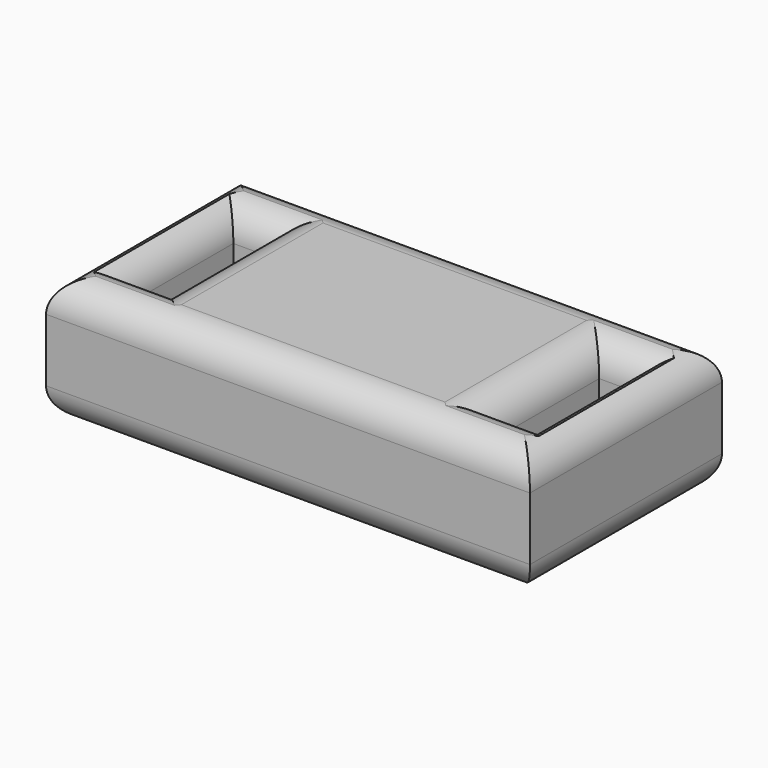
from build123d import *

# Parameters (mm, degrees)
F0_W          = 30.75
F0_H          = 15.25
F0_W_2        = 2.5
F0_H_2        = 8.25
F1_DEPTH      = 8
F2_T1_DEPTH   = 40.75
F2_T3_DEPTH   = 25.25
F2_T5_DEPTH   = 2.5
F2_T7_DEPTH   = 8.25
F2_T9_DEPTH   = 2.5
F2_T15_DEPTH  = 7.5
F2_T20_DEPTH  = 13.25
F2_T28_DEPTH  = 7.5
F2_T32_DEPTH  = 13.25
F2_T40_DEPTH  = 13.25
F2_T45_DEPTH  = 7.5
F2_T52_DEPTH  = 7.5
F2_T57_DEPTH  = 13.25
F2_T65_DEPTH  = 13.25
F2_T70_DEPTH  = 7.5
F2_T77_DEPTH  = 13.25
F2_T82_DEPTH  = 7.5
F2_T89_DEPTH  = 7.5
F2_T94_DEPTH  = 13.25
F2_T102_DEPTH = 13.25
F2_T107_DEPTH = 7.5
F2_T115_DEPTH = 7.5
F2_T120_DEPTH = 13.25
F2_T128_DEPTH = 7.5
F2_T132_DEPTH = 13.25
F2_T140_DEPTH = 13.25
F2_T145_DEPTH = 7.5
F2_T152_DEPTH = 7.5
F2_T157_DEPTH = 13.25
F2_T165_DEPTH = 13.25
F2_T170_DEPTH = 7.5
F2_T177_DEPTH = 13.25
F2_T182_DEPTH = 7.5
F2_T189_DEPTH = 7.5
F2_T194_DEPTH = 13.25
F2_T202_DEPTH = 13.25
F2_T207_DEPTH = 7.5


# Not quite as in the source:
# - a fillet or chamfer that OpenCascade refuses, or shapes differently, is made with other operations: its cross-section is extruded or revolved along the edge and cut away or added


with BuildPart() as f1:
    # F0 (on Top) → F1 (new body)
    with BuildSketch(Plane.XY):
        Rectangle(F0_W, F0_H)
        with Locations((-11.625, 0)):
            Rectangle(F0_W_2, F0_H_2, mode=Mode.SUBTRACT)
        with Locations((11.625, 0)):
            Rectangle(F0_W_2, F0_H_2, mode=Mode.SUBTRACT)
    extrude(amount=F1_DEPTH)

    # F2: fillet of radius 2 on 24 edges, made by hand

    # F2_s2 → F2_t1 (cut)
    with BuildSketch(Plane.YZ.offset(-20.375)):
        with BuildLine():
            ThreePointArc((7.625, 6), (7.0392135624, 7.4142135624), (5.625, 8))
            Line((5.625, 8), (7.625, 8))
            Line((7.625, 8), (7.625, 6))
        make_face()
        with BuildLine():
            ThreePointArc((-7.625, 6), (-7.0392135624, 7.4142135624), (-5.625, 8))
            Line((-5.625, 8), (-7.625, 8))
            Line((-7.625, 8), (-7.625, 6))
        make_face()
        with BuildLine():
            ThreePointArc((7.625, 2), (7.0392135624, 0.5857864376), (5.625, 0))
            Line((5.625, 0), (7.625, 0))
            Line((7.625, 0), (7.625, 2))
        make_face()
        with BuildLine():
            ThreePointArc((-7.625, 2), (-7.0392135624, 0.5857864376), (-5.625, 0))
            Line((-5.625, 0), (-7.625, 0))
            Line((-7.625, 0), (-7.625, 2))
        make_face()
    extrude(amount=F2_T1_DEPTH, mode=Mode.SUBTRACT)

    # F2_s4 → F2_t3 (cut)
    with BuildSketch(Plane.XZ.offset(-12.625)):
        with BuildLine():
            ThreePointArc((-15.375, 6), (-14.7892135624, 7.4142135624), (-13.375, 8))
            Line((-13.375, 8), (-15.375, 8))
            Line((-15.375, 8), (-15.375, 6))
        make_face()
        with BuildLine():
            ThreePointArc((15.375, 6), (14.7892135624, 7.4142135624), (13.375, 8))
            Line((13.375, 8), (15.375, 8))
            Line((15.375, 8), (15.375, 6))
        make_face()
        with BuildLine():
            ThreePointArc((-15.375, 2), (-14.7892135624, 0.5857864376), (-13.375, 0))
            Line((-13.375, 0), (-15.375, 0))
            Line((-15.375, 0), (-15.375, 2))
        make_face()
        with BuildLine():
            ThreePointArc((15.375, 2), (14.7892135624, 0.5857864376), (13.375, 0))
            Line((13.375, 0), (15.375, 0))
            Line((15.375, 0), (15.375, 2))
        make_face()
    extrude(amount=F2_T3_DEPTH, mode=Mode.SUBTRACT)

    # F2_s6 → F2_t5 (cut)
    with BuildSketch(Plane.YZ.offset(-12.875)):
        with BuildLine():
            ThreePointArc((4.125, 6), (4.7107864376, 7.4142135624), (6.125, 8))
            Line((6.125, 8), (4.125, 8))
            Line((4.125, 8), (4.125, 6))
        make_face()
        with BuildLine():
            ThreePointArc((-4.125, 6), (-4.7107864376, 7.4142135624), (-6.125, 8))
            Line((-6.125, 8), (-4.125, 8))
            Line((-4.125, 8), (-4.125, 6))
        make_face()
        with BuildLine():
            ThreePointArc((4.125, 2), (4.7107864376, 0.5857864376), (6.125, 0))
            Line((6.125, 0), (4.125, 0))
            Line((4.125, 0), (4.125, 2))
        make_face()
        with BuildLine():
            ThreePointArc((-4.125, 2), (-4.7107864376, 0.5857864376), (-6.125, 0))
            Line((-6.125, 0), (-4.125, 0))
            Line((-4.125, 0), (-4.125, 2))
        make_face()
    extrude(amount=F2_T5_DEPTH, mode=Mode.SUBTRACT)

    # F2_s8 → F2_t7 (cut)
    with BuildSketch(Plane.XZ.offset(-4.125)):
        with BuildLine():
            ThreePointArc((-10.375, 6), (-9.7892135624, 7.4142135624), (-8.375, 8))
            Line((-8.375, 8), (-10.375, 8))
            Line((-10.375, 8), (-10.375, 6))
        make_face()
        with BuildLine():
            ThreePointArc((-12.875, 6), (-13.4607864376, 7.4142135624), (-14.875, 8))
            Line((-14.875, 8), (-12.875, 8))
            Line((-12.875, 8), (-12.875, 6))
        make_face()
        with BuildLine():
            ThreePointArc((10.375, 6), (9.7892135624, 7.4142135624), (8.375, 8))
            Line((8.375, 8), (10.375, 8))
            Line((10.375, 8), (10.375, 6))
        make_face()
        with BuildLine():
            ThreePointArc((12.875, 6), (13.4607864376, 7.4142135624), (14.875, 8))
            Line((14.875, 8), (12.875, 8))
            Line((12.875, 8), (12.875, 6))
        make_face()
        with BuildLine():
            ThreePointArc((-10.375, 2), (-9.7892135624, 0.5857864376), (-8.375, 0))
            Line((-8.375, 0), (-10.375, 0))
            Line((-10.375, 0), (-10.375, 2))
        make_face()
        with BuildLine():
            ThreePointArc((-12.875, 2), (-13.4607864376, 0.5857864376), (-14.875, 0))
            Line((-14.875, 0), (-12.875, 0))
            Line((-12.875, 0), (-12.875, 2))
        make_face()
        with BuildLine():
            ThreePointArc((10.375, 2), (9.7892135624, 0.5857864376), (8.375, 0))
            Line((8.375, 0), (10.375, 0))
            Line((10.375, 0), (10.375, 2))
        make_face()
        with BuildLine():
            ThreePointArc((12.875, 2), (13.4607864376, 0.5857864376), (14.875, 0))
            Line((14.875, 0), (12.875, 0))
            Line((12.875, 0), (12.875, 2))
        make_face()
    extrude(amount=F2_T7_DEPTH, mode=Mode.SUBTRACT)

    # F2_s10 → F2_t9 (cut)
    with BuildSketch(Plane.YZ.offset(10.375)):
        with BuildLine():
            ThreePointArc((4.125, 6), (4.7107864376, 7.4142135624), (6.125, 8))
            Line((6.125, 8), (4.125, 8))
            Line((4.125, 8), (4.125, 6))
        make_face()
        with BuildLine():
            ThreePointArc((-4.125, 6), (-4.7107864376, 7.4142135624), (-6.125, 8))
            Line((-6.125, 8), (-4.125, 8))
            Line((-4.125, 8), (-4.125, 6))
        make_face()
        with BuildLine():
            ThreePointArc((4.125, 2), (4.7107864376, 0.5857864376), (6.125, 0))
            Line((6.125, 0), (4.125, 0))
            Line((4.125, 0), (4.125, 2))
        make_face()
        with BuildLine():
            ThreePointArc((-4.125, 2), (-4.7107864376, 0.5857864376), (-6.125, 0))
            Line((-6.125, 0), (-4.125, 0))
            Line((-4.125, 0), (-4.125, 2))
        make_face()
    extrude(amount=F2_T9_DEPTH, mode=Mode.SUBTRACT)


with BuildPart() as f2_tool13:
    # F2_s14 → F2_t15 (new body)
    with BuildSketch(Plane.YZ.offset(-17.875)):
        with BuildLine():
            ThreePointArc((4.125, 6), (4.7107864376, 7.4142135624), (6.125, 8))
            Line((6.125, 8), (4.125, 8))
            Line((4.125, 8), (4.125, 6))
        make_face()
    extrude(amount=F2_T15_DEPTH)

    split(bisect_by=Plane.YZ.offset(-15.375), keep=Keep.TOP)

    split(bisect_by=Plane.YZ.offset(-12.875), keep=Keep.BOTTOM)


with BuildPart() as f2_tool18:
    # F2_s19 → F2_t20 (new body)
    with BuildSketch(Plane.XZ.offset(4.125)):
        with BuildLine():
            ThreePointArc((-12.875, 6), (-13.4607864376, 7.4142135624), (-14.875, 8))
            Line((-14.875, 8), (-12.875, 8))
            Line((-12.875, 8), (-12.875, 6))
        make_face()
    extrude(amount=-F2_T20_DEPTH)

    split(bisect_by=Plane.XZ.offset(-7.625), keep=Keep.TOP)

    split(bisect_by=Plane.XZ.offset(-4.125), keep=Keep.BOTTOM)


with BuildPart() as f2_tool13_1:
    add(f2_tool13.part)

    # F2_t23: intersect F2_tool18
    add(f2_tool18.part, mode=Mode.INTERSECT)


with BuildPart() as f1_1:
    add(f1.part)

    # F2_t11: cut F2_tool13
    add(f2_tool13_1.part, mode=Mode.SUBTRACT)


with BuildPart() as f2_tool26:
    # F2_s27 → F2_t28 (new body)
    with BuildSketch(Plane.YZ.offset(-12.875)):
        with BuildLine():
            ThreePointArc((4.125, 6), (4.7107864376, 7.4142135624), (6.125, 8))
            Line((6.125, 8), (4.125, 8))
            Line((4.125, 8), (4.125, 6))
        make_face()
    extrude(amount=F2_T28_DEPTH)

    split(bisect_by=Plane.YZ.offset(-10.375), keep=Keep.TOP)


with BuildPart() as f2_tool30:
    # F2_s31 → F2_t32 (new body)
    with BuildSketch(Plane.XZ.offset(-9.125)):
        with BuildLine():
            ThreePointArc((-10.375, 6), (-9.7892135624, 7.4142135624), (-8.375, 8))
            Line((-8.375, 8), (-10.375, 8))
            Line((-10.375, 8), (-10.375, 6))
        make_face()
    extrude(amount=F2_T32_DEPTH)

    split(bisect_by=Plane.XZ.offset(-7.625), keep=Keep.TOP)

    split(bisect_by=Plane.XZ.offset(-4.125), keep=Keep.BOTTOM)


with BuildPart() as f2_tool26_1:
    add(f2_tool26.part)

    # F2_t35: intersect F2_tool30
    add(f2_tool30.part, mode=Mode.INTERSECT)


with BuildPart() as f1_2:
    add(f1_1.part)

    # F2_t24: cut F2_tool26
    add(f2_tool26_1.part, mode=Mode.SUBTRACT)


with BuildPart() as f2_tool38:
    # F2_s39 → F2_t40 (new body)
    with BuildSketch(Plane.XZ.offset(-4.125)):
        with BuildLine():
            ThreePointArc((-10.375, 6), (-9.7892135624, 7.4142135624), (-8.375, 8))
            Line((-8.375, 8), (-10.375, 8))
            Line((-10.375, 8), (-10.375, 6))
        make_face()
    extrude(amount=F2_T40_DEPTH)

    split(bisect_by=Plane.XZ.offset(7.625), keep=Keep.BOTTOM)

    split(bisect_by=Plane.XZ.offset(4.125), keep=Keep.TOP)


with BuildPart() as f2_tool43:
    # F2_s44 → F2_t45 (new body)
    with BuildSketch(Plane.YZ.offset(-5.375)):
        with BuildLine():
            ThreePointArc((-4.125, 6), (-4.7107864376, 7.4142135624), (-6.125, 8))
            Line((-6.125, 8), (-4.125, 8))
            Line((-4.125, 8), (-4.125, 6))
        make_face()
    extrude(amount=-F2_T45_DEPTH)

    split(bisect_by=Plane.YZ.offset(-10.375), keep=Keep.TOP)


with BuildPart() as f2_tool38_1:
    add(f2_tool38.part)

    # F2_t47: intersect F2_tool43
    add(f2_tool43.part, mode=Mode.INTERSECT)


with BuildPart() as f1_3:
    add(f1_2.part)

    # F2_t36: cut F2_tool38
    add(f2_tool38_1.part, mode=Mode.SUBTRACT)


with BuildPart() as f2_tool50:
    # F2_s51 → F2_t52 (new body)
    with BuildSketch(Plane.YZ.offset(-10.375)):
        with BuildLine():
            ThreePointArc((-4.125, 6), (-4.7107864376, 7.4142135624), (-6.125, 8))
            Line((-6.125, 8), (-4.125, 8))
            Line((-4.125, 8), (-4.125, 6))
        make_face()
    extrude(amount=-F2_T52_DEPTH)

    split(bisect_by=Plane.YZ.offset(-15.375), keep=Keep.TOP)

    split(bisect_by=Plane.YZ.offset(-12.875), keep=Keep.BOTTOM)


with BuildPart() as f2_tool55:
    # F2_s56 → F2_t57 (new body)
    with BuildSketch(Plane.XZ.offset(9.125)):
        with BuildLine():
            ThreePointArc((-12.875, 6), (-13.4607864376, 7.4142135624), (-14.875, 8))
            Line((-14.875, 8), (-12.875, 8))
            Line((-12.875, 8), (-12.875, 6))
        make_face()
    extrude(amount=-F2_T57_DEPTH)

    split(bisect_by=Plane.XZ.offset(7.625), keep=Keep.BOTTOM)

    split(bisect_by=Plane.XZ.offset(4.125), keep=Keep.TOP)


with BuildPart() as f2_tool50_1:
    add(f2_tool50.part)

    # F2_t60: intersect F2_tool55
    add(f2_tool55.part, mode=Mode.INTERSECT)


with BuildPart() as f1_4:
    add(f1_3.part)

    # F2_t48: cut F2_tool50
    add(f2_tool50_1.part, mode=Mode.SUBTRACT)


with BuildPart() as f2_tool63:
    # F2_s64 → F2_t65 (new body)
    with BuildSketch(Plane.XZ.offset(9.125)):
        with BuildLine():
            ThreePointArc((10.375, 6), (9.7892135624, 7.4142135624), (8.375, 8))
            Line((8.375, 8), (10.375, 8))
            Line((10.375, 8), (10.375, 6))
        make_face()
    extrude(amount=-F2_T65_DEPTH)

    split(bisect_by=Plane.XZ.offset(7.625), keep=Keep.BOTTOM)

    split(bisect_by=Plane.XZ.offset(4.125), keep=Keep.TOP)


with BuildPart() as f2_tool68:
    # F2_s69 → F2_t70 (new body)
    with BuildSketch(Plane.YZ.offset(12.875)):
        with BuildLine():
            ThreePointArc((-4.125, 6), (-4.7107864376, 7.4142135624), (-6.125, 8))
            Line((-6.125, 8), (-4.125, 8))
            Line((-4.125, 8), (-4.125, 6))
        make_face()
    extrude(amount=-F2_T70_DEPTH)

    split(bisect_by=Plane.YZ.offset(10.375), keep=Keep.BOTTOM)


with BuildPart() as f2_tool63_1:
    add(f2_tool63.part)

    # F2_t72: intersect F2_tool68
    add(f2_tool68.part, mode=Mode.INTERSECT)


with BuildPart() as f1_5:
    add(f1_4.part)

    # F2_t61: cut F2_tool63
    add(f2_tool63_1.part, mode=Mode.SUBTRACT)


with BuildPart() as f2_tool75:
    # F2_s76 → F2_t77 (new body)
    with BuildSketch(Plane.XZ.offset(4.125)):
        with BuildLine():
            ThreePointArc((10.375, 6), (9.7892135624, 7.4142135624), (8.375, 8))
            Line((8.375, 8), (10.375, 8))
            Line((10.375, 8), (10.375, 6))
        make_face()
    extrude(amount=-F2_T77_DEPTH)

    split(bisect_by=Plane.XZ.offset(-7.625), keep=Keep.TOP)

    split(bisect_by=Plane.XZ.offset(-4.125), keep=Keep.BOTTOM)


with BuildPart() as f2_tool80:
    # F2_s81 → F2_t82 (new body)
    with BuildSketch(Plane.YZ.offset(5.375)):
        with BuildLine():
            ThreePointArc((4.125, 6), (4.7107864376, 7.4142135624), (6.125, 8))
            Line((6.125, 8), (4.125, 8))
            Line((4.125, 8), (4.125, 6))
        make_face()
    extrude(amount=F2_T82_DEPTH)

    split(bisect_by=Plane.YZ.offset(10.375), keep=Keep.BOTTOM)


with BuildPart() as f2_tool75_1:
    add(f2_tool75.part)

    # F2_t84: intersect F2_tool80
    add(f2_tool80.part, mode=Mode.INTERSECT)


with BuildPart() as f1_6:
    add(f1_5.part)

    # F2_t73: cut F2_tool75
    add(f2_tool75_1.part, mode=Mode.SUBTRACT)


with BuildPart() as f2_tool87:
    # F2_s88 → F2_t89 (new body)
    with BuildSketch(Plane.YZ.offset(10.375)):
        with BuildLine():
            ThreePointArc((4.125, 6), (4.7107864376, 7.4142135624), (6.125, 8))
            Line((6.125, 8), (4.125, 8))
            Line((4.125, 8), (4.125, 6))
        make_face()
    extrude(amount=F2_T89_DEPTH)

    split(bisect_by=Plane.YZ.offset(15.375), keep=Keep.BOTTOM)

    split(bisect_by=Plane.YZ.offset(12.875), keep=Keep.TOP)


with BuildPart() as f2_tool92:
    # F2_s93 → F2_t94 (new body)
    with BuildSketch(Plane.XZ.offset(-9.125)):
        with BuildLine():
            ThreePointArc((12.875, 6), (13.4607864376, 7.4142135624), (14.875, 8))
            Line((14.875, 8), (12.875, 8))
            Line((12.875, 8), (12.875, 6))
        make_face()
    extrude(amount=F2_T94_DEPTH)

    split(bisect_by=Plane.XZ.offset(-7.625), keep=Keep.TOP)

    split(bisect_by=Plane.XZ.offset(-4.125), keep=Keep.BOTTOM)


with BuildPart() as f2_tool87_1:
    add(f2_tool87.part)

    # F2_t97: intersect F2_tool92
    add(f2_tool92.part, mode=Mode.INTERSECT)


with BuildPart() as f1_7:
    add(f1_6.part)

    # F2_t85: cut F2_tool87
    add(f2_tool87_1.part, mode=Mode.SUBTRACT)


with BuildPart() as f2_tool100:
    # F2_s101 → F2_t102 (new body)
    with BuildSketch(Plane.XZ.offset(-4.125)):
        with BuildLine():
            ThreePointArc((12.875, 6), (13.4607864376, 7.4142135624), (14.875, 8))
            Line((14.875, 8), (12.875, 8))
            Line((12.875, 8), (12.875, 6))
        make_face()
    extrude(amount=F2_T102_DEPTH)

    split(bisect_by=Plane.XZ.offset(7.625), keep=Keep.BOTTOM)

    split(bisect_by=Plane.XZ.offset(4.125), keep=Keep.TOP)


with BuildPart() as f2_tool105:
    # F2_s106 → F2_t107 (new body)
    with BuildSketch(Plane.YZ.offset(17.875)):
        with BuildLine():
            ThreePointArc((-4.125, 6), (-4.7107864376, 7.4142135624), (-6.125, 8))
            Line((-6.125, 8), (-4.125, 8))
            Line((-4.125, 8), (-4.125, 6))
        make_face()
    extrude(amount=-F2_T107_DEPTH)

    split(bisect_by=Plane.YZ.offset(15.375), keep=Keep.BOTTOM)

    split(bisect_by=Plane.YZ.offset(12.875), keep=Keep.TOP)


with BuildPart() as f2_tool100_1:
    add(f2_tool100.part)

    # F2_t110: intersect F2_tool105
    add(f2_tool105.part, mode=Mode.INTERSECT)


with BuildPart() as f1_8:
    add(f1_7.part)

    # F2_t98: cut F2_tool100
    add(f2_tool100_1.part, mode=Mode.SUBTRACT)


with BuildPart() as f2_tool113:
    # F2_s114 → F2_t115 (new body)
    with BuildSketch(Plane.YZ.offset(-17.875)):
        with BuildLine():
            ThreePointArc((4.125, 2), (4.7107864376, 0.5857864376), (6.125, 0))
            Line((6.125, 0), (4.125, 0))
            Line((4.125, 0), (4.125, 2))
        make_face()
    extrude(amount=F2_T115_DEPTH)

    split(bisect_by=Plane.YZ.offset(-15.375), keep=Keep.TOP)

    split(bisect_by=Plane.YZ.offset(-12.875), keep=Keep.BOTTOM)


with BuildPart() as f2_tool118:
    # F2_s119 → F2_t120 (new body)
    with BuildSketch(Plane.XZ.offset(4.125)):
        with BuildLine():
            ThreePointArc((-12.875, 2), (-13.4607864376, 0.5857864376), (-14.875, 0))
            Line((-14.875, 0), (-12.875, 0))
            Line((-12.875, 0), (-12.875, 2))
        make_face()
    extrude(amount=-F2_T120_DEPTH)

    split(bisect_by=Plane.XZ.offset(-7.625), keep=Keep.TOP)

    split(bisect_by=Plane.XZ.offset(-4.125), keep=Keep.BOTTOM)


with BuildPart() as f2_tool113_1:
    add(f2_tool113.part)

    # F2_t123: intersect F2_tool118
    add(f2_tool118.part, mode=Mode.INTERSECT)


with BuildPart() as f1_9:
    add(f1_8.part)

    # F2_t111: cut F2_tool113
    add(f2_tool113_1.part, mode=Mode.SUBTRACT)


with BuildPart() as f2_tool126:
    # F2_s127 → F2_t128 (new body)
    with BuildSketch(Plane.YZ.offset(-12.875)):
        with BuildLine():
            ThreePointArc((4.125, 2), (4.7107864376, 0.5857864376), (6.125, 0))
            Line((6.125, 0), (4.125, 0))
            Line((4.125, 0), (4.125, 2))
        make_face()
    extrude(amount=F2_T128_DEPTH)

    split(bisect_by=Plane.YZ.offset(-10.375), keep=Keep.TOP)


with BuildPart() as f2_tool130:
    # F2_s131 → F2_t132 (new body)
    with BuildSketch(Plane.XZ.offset(-9.125)):
        with BuildLine():
            ThreePointArc((-10.375, 2), (-9.7892135624, 0.5857864376), (-8.375, 0))
            Line((-8.375, 0), (-10.375, 0))
            Line((-10.375, 0), (-10.375, 2))
        make_face()
    extrude(amount=F2_T132_DEPTH)

    split(bisect_by=Plane.XZ.offset(-7.625), keep=Keep.TOP)

    split(bisect_by=Plane.XZ.offset(-4.125), keep=Keep.BOTTOM)


with BuildPart() as f2_tool126_1:
    add(f2_tool126.part)

    # F2_t135: intersect F2_tool130
    add(f2_tool130.part, mode=Mode.INTERSECT)


with BuildPart() as f1_10:
    add(f1_9.part)

    # F2_t124: cut F2_tool126
    add(f2_tool126_1.part, mode=Mode.SUBTRACT)


with BuildPart() as f2_tool138:
    # F2_s139 → F2_t140 (new body)
    with BuildSketch(Plane.XZ.offset(-4.125)):
        with BuildLine():
            ThreePointArc((-10.375, 2), (-9.7892135624, 0.5857864376), (-8.375, 0))
            Line((-8.375, 0), (-10.375, 0))
            Line((-10.375, 0), (-10.375, 2))
        make_face()
    extrude(amount=F2_T140_DEPTH)

    split(bisect_by=Plane.XZ.offset(7.625), keep=Keep.BOTTOM)

    split(bisect_by=Plane.XZ.offset(4.125), keep=Keep.TOP)


with BuildPart() as f2_tool143:
    # F2_s144 → F2_t145 (new body)
    with BuildSketch(Plane.YZ.offset(-5.375)):
        with BuildLine():
            ThreePointArc((-4.125, 2), (-4.7107864376, 0.5857864376), (-6.125, 0))
            Line((-6.125, 0), (-4.125, 0))
            Line((-4.125, 0), (-4.125, 2))
        make_face()
    extrude(amount=-F2_T145_DEPTH)

    split(bisect_by=Plane.YZ.offset(-10.375), keep=Keep.TOP)


with BuildPart() as f2_tool138_1:
    add(f2_tool138.part)

    # F2_t147: intersect F2_tool143
    add(f2_tool143.part, mode=Mode.INTERSECT)


with BuildPart() as f1_11:
    add(f1_10.part)

    # F2_t136: cut F2_tool138
    add(f2_tool138_1.part, mode=Mode.SUBTRACT)


with BuildPart() as f2_tool150:
    # F2_s151 → F2_t152 (new body)
    with BuildSketch(Plane.YZ.offset(-10.375)):
        with BuildLine():
            ThreePointArc((-4.125, 2), (-4.7107864376, 0.5857864376), (-6.125, 0))
            Line((-6.125, 0), (-4.125, 0))
            Line((-4.125, 0), (-4.125, 2))
        make_face()
    extrude(amount=-F2_T152_DEPTH)

    split(bisect_by=Plane.YZ.offset(-15.375), keep=Keep.TOP)

    split(bisect_by=Plane.YZ.offset(-12.875), keep=Keep.BOTTOM)


with BuildPart() as f2_tool155:
    # F2_s156 → F2_t157 (new body)
    with BuildSketch(Plane.XZ.offset(9.125)):
        with BuildLine():
            ThreePointArc((-12.875, 2), (-13.4607864376, 0.5857864376), (-14.875, 0))
            Line((-14.875, 0), (-12.875, 0))
            Line((-12.875, 0), (-12.875, 2))
        make_face()
    extrude(amount=-F2_T157_DEPTH)

    split(bisect_by=Plane.XZ.offset(7.625), keep=Keep.BOTTOM)

    split(bisect_by=Plane.XZ.offset(4.125), keep=Keep.TOP)


with BuildPart() as f2_tool150_1:
    add(f2_tool150.part)

    # F2_t160: intersect F2_tool155
    add(f2_tool155.part, mode=Mode.INTERSECT)


with BuildPart() as f1_12:
    add(f1_11.part)

    # F2_t148: cut F2_tool150
    add(f2_tool150_1.part, mode=Mode.SUBTRACT)


with BuildPart() as f2_tool163:
    # F2_s164 → F2_t165 (new body)
    with BuildSketch(Plane.XZ.offset(9.125)):
        with BuildLine():
            ThreePointArc((10.375, 2), (9.7892135624, 0.5857864376), (8.375, 0))
            Line((8.375, 0), (10.375, 0))
            Line((10.375, 0), (10.375, 2))
        make_face()
    extrude(amount=-F2_T165_DEPTH)

    split(bisect_by=Plane.XZ.offset(7.625), keep=Keep.BOTTOM)

    split(bisect_by=Plane.XZ.offset(4.125), keep=Keep.TOP)


with BuildPart() as f2_tool168:
    # F2_s169 → F2_t170 (new body)
    with BuildSketch(Plane.YZ.offset(12.875)):
        with BuildLine():
            ThreePointArc((-4.125, 2), (-4.7107864376, 0.5857864376), (-6.125, 0))
            Line((-6.125, 0), (-4.125, 0))
            Line((-4.125, 0), (-4.125, 2))
        make_face()
    extrude(amount=-F2_T170_DEPTH)

    split(bisect_by=Plane.YZ.offset(10.375), keep=Keep.BOTTOM)


with BuildPart() as f2_tool163_1:
    add(f2_tool163.part)

    # F2_t172: intersect F2_tool168
    add(f2_tool168.part, mode=Mode.INTERSECT)


with BuildPart() as f1_13:
    add(f1_12.part)

    # F2_t161: cut F2_tool163
    add(f2_tool163_1.part, mode=Mode.SUBTRACT)


with BuildPart() as f2_tool175:
    # F2_s176 → F2_t177 (new body)
    with BuildSketch(Plane.XZ.offset(4.125)):
        with BuildLine():
            ThreePointArc((10.375, 2), (9.7892135624, 0.5857864376), (8.375, 0))
            Line((8.375, 0), (10.375, 0))
            Line((10.375, 0), (10.375, 2))
        make_face()
    extrude(amount=-F2_T177_DEPTH)

    split(bisect_by=Plane.XZ.offset(-7.625), keep=Keep.TOP)

    split(bisect_by=Plane.XZ.offset(-4.125), keep=Keep.BOTTOM)


with BuildPart() as f2_tool180:
    # F2_s181 → F2_t182 (new body)
    with BuildSketch(Plane.YZ.offset(5.375)):
        with BuildLine():
            ThreePointArc((4.125, 2), (4.7107864376, 0.5857864376), (6.125, 0))
            Line((6.125, 0), (4.125, 0))
            Line((4.125, 0), (4.125, 2))
        make_face()
    extrude(amount=F2_T182_DEPTH)

    split(bisect_by=Plane.YZ.offset(10.375), keep=Keep.BOTTOM)


with BuildPart() as f2_tool175_1:
    add(f2_tool175.part)

    # F2_t184: intersect F2_tool180
    add(f2_tool180.part, mode=Mode.INTERSECT)


with BuildPart() as f1_14:
    add(f1_13.part)

    # F2_t173: cut F2_tool175
    add(f2_tool175_1.part, mode=Mode.SUBTRACT)


with BuildPart() as f2_tool187:
    # F2_s188 → F2_t189 (new body)
    with BuildSketch(Plane.YZ.offset(10.375)):
        with BuildLine():
            ThreePointArc((4.125, 2), (4.7107864376, 0.5857864376), (6.125, 0))
            Line((6.125, 0), (4.125, 0))
            Line((4.125, 0), (4.125, 2))
        make_face()
    extrude(amount=F2_T189_DEPTH)

    split(bisect_by=Plane.YZ.offset(15.375), keep=Keep.BOTTOM)

    split(bisect_by=Plane.YZ.offset(12.875), keep=Keep.TOP)


with BuildPart() as f2_tool192:
    # F2_s193 → F2_t194 (new body)
    with BuildSketch(Plane.XZ.offset(-9.125)):
        with BuildLine():
            ThreePointArc((12.875, 2), (13.4607864376, 0.5857864376), (14.875, 0))
            Line((14.875, 0), (12.875, 0))
            Line((12.875, 0), (12.875, 2))
        make_face()
    extrude(amount=F2_T194_DEPTH)

    split(bisect_by=Plane.XZ.offset(-7.625), keep=Keep.TOP)

    split(bisect_by=Plane.XZ.offset(-4.125), keep=Keep.BOTTOM)


with BuildPart() as f2_tool187_1:
    add(f2_tool187.part)

    # F2_t197: intersect F2_tool192
    add(f2_tool192.part, mode=Mode.INTERSECT)


with BuildPart() as f1_15:
    add(f1_14.part)

    # F2_t185: cut F2_tool187
    add(f2_tool187_1.part, mode=Mode.SUBTRACT)


with BuildPart() as f2_tool200:
    # F2_s201 → F2_t202 (new body)
    with BuildSketch(Plane.XZ.offset(-4.125)):
        with BuildLine():
            ThreePointArc((12.875, 2), (13.4607864376, 0.5857864376), (14.875, 0))
            Line((14.875, 0), (12.875, 0))
            Line((12.875, 0), (12.875, 2))
        make_face()
    extrude(amount=F2_T202_DEPTH)

    split(bisect_by=Plane.XZ.offset(7.625), keep=Keep.BOTTOM)

    split(bisect_by=Plane.XZ.offset(4.125), keep=Keep.TOP)


with BuildPart() as f2_tool205:
    # F2_s206 → F2_t207 (new body)
    with BuildSketch(Plane.YZ.offset(17.875)):
        with BuildLine():
            ThreePointArc((-4.125, 2), (-4.7107864376, 0.5857864376), (-6.125, 0))
            Line((-6.125, 0), (-4.125, 0))
            Line((-4.125, 0), (-4.125, 2))
        make_face()
    extrude(amount=-F2_T207_DEPTH)

    split(bisect_by=Plane.YZ.offset(15.375), keep=Keep.BOTTOM)

    split(bisect_by=Plane.YZ.offset(12.875), keep=Keep.TOP)


with BuildPart() as f2_tool200_1:
    add(f2_tool200.part)

    # F2_t210: intersect F2_tool205
    add(f2_tool205.part, mode=Mode.INTERSECT)


with BuildPart() as f1_16:
    add(f1_15.part)

    # F2_t198: cut F2_tool200
    add(f2_tool200_1.part, mode=Mode.SUBTRACT)


solid = f1_16.part
